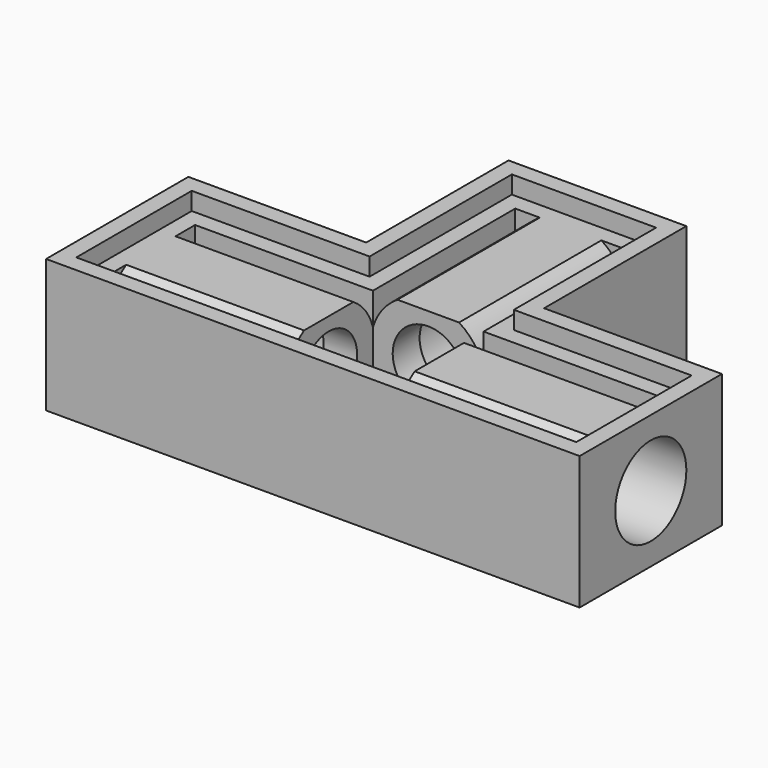
from build123d import *

# Parameters (mm, degrees)
F1_DEPTH  = 19.05
F2_T      = -2.4
F4_DEPTH  = 14.11
F5_R      = 8.255
F5_R_2    = 6.35
F5_R_3    = 5.08
F6_DEPTH  = 30.2
F7_DEPTH  = 25.4
F8_DEPTH  = 34.5948
F9_R      = 8.255
F9_R_2    = 6.35
F9_R_3    = 5.08
F10_DEPTH = 30.2
F11_DEPTH = 25.4
F12_DEPTH = 36.9316
F13_R     = 8.255
F13_R_2   = 6.35
F13_R_3   = 5.08
F14_DEPTH = 30.2
F15_DEPTH = 25.4
F16_DEPTH = 31.242
F17_W     = 3.7311392443
F17_H     = 25.4
F17_W_2   = 25.4
F17_H_2   = 3.7311392443
F20_DEPTH = 2.54


with BuildPart() as f1:
    # F0 (on Top) → F1 (new body)
    with BuildSketch(Plane.XY):
        Polygon((-12.7, 25.4), (-38.1, 25.4), (-38.1, 0), (38.1, 0), (38.1, 25.4), (12.7, 25.4), (12.7, 50.8), (-12.7, 50.8), align=None)
    extrude(amount=F1_DEPTH)

    # F2
    f2_openings = [f1.faces().sort_by_distance(p)[0] for p in [
        (0, 19.05, 19.05),
    ]]
    offset(amount=F2_T, openings=f2_openings, kind=Kind.INTERSECTION)

    # F3 (on face) → F4 (join, through all)
    with BuildSketch(Plane.XY.offset(2.4)):
        Polygon((10.3, 48.4), (-10.3, 48.4), (-10.3, 23), (-35.7, 23), (-35.7, 2.4), (35.7, 2.4), (35.7, 23), (10.3, 23), align=None)
        Polygon((-33.3, 4.8), (-33.3, 20.6), (-7.9, 20.6), (-7.9, 46), (7.9, 46), (7.9, 20.6), (33.3, 20.6), (33.3, 4.8), align=None, mode=Mode.SUBTRACT)
    extrude(amount=F4_DEPTH)

    # F5 (on face) → F6 (join, through all)
    with BuildSketch(Plane(origin=(0, 50.8, 0), x_dir=(-1, 0, 0), z_dir=(0, 1, 0))):
        with Locations((0, 9.525)):
            Circle(F5_R)
        with Locations((0, 9.525)):
            Circle(F5_R_2, mode=Mode.SUBTRACT)
        with Locations((0, 9.525)):
            Circle(F5_R_2)
        with Locations((0, 9.525)):
            Circle(F5_R_3, mode=Mode.SUBTRACT)
        with Locations((0, 9.525)):
            Circle(F5_R_3)
    extrude(amount=-F6_DEPTH)

    # F5 (on face) → F7 (cut)
    with BuildSketch(Plane(origin=(0, 50.8, 0), x_dir=(-1, 0, 0), z_dir=(0, 1, 0))):
        with Locations((0, 9.525)):
            Circle(F5_R_2)
        with Locations((0, 9.525)):
            Circle(F5_R_3, mode=Mode.SUBTRACT)
        with Locations((0, 9.525)):
            Circle(F5_R_3)
    extrude(amount=-F7_DEPTH, mode=Mode.SUBTRACT)

    # F5 (on face) → F8 (cut)
    with BuildSketch(Plane(origin=(0, 50.8, 0), x_dir=(-1, 0, 0), z_dir=(0, 1, 0))):
        with Locations((0, 9.525)):
            Circle(F5_R_3)
    extrude(amount=-F8_DEPTH, mode=Mode.SUBTRACT)

    # F9 (on face) → F10 (join, through all)
    with BuildSketch(Plane.YZ.offset(38.1)):
        with Locations((12.7, 9.525)):
            Circle(F9_R)
        with Locations((12.7, 9.525)):
            Circle(F9_R_2, mode=Mode.SUBTRACT)
        with Locations((12.7, 9.525)):
            Circle(F9_R_2)
        with Locations((12.7, 9.525)):
            Circle(F9_R_3, mode=Mode.SUBTRACT)
        with Locations((12.7, 9.525)):
            Circle(F9_R_3)
    extrude(amount=-F10_DEPTH)

    # F9 (on face) → F11 (cut)
    with BuildSketch(Plane.YZ.offset(38.1)):
        with Locations((12.7, 9.525)):
            Circle(F9_R_2)
        with Locations((12.7, 9.525)):
            Circle(F9_R_3, mode=Mode.SUBTRACT)
    extrude(amount=-F11_DEPTH, mode=Mode.SUBTRACT)

    # F9 (on face) → F12 (cut)
    with BuildSketch(Plane.YZ.offset(38.1)):
        with Locations((12.7, 9.525)):
            Circle(F9_R_3)
    extrude(amount=-F12_DEPTH, mode=Mode.SUBTRACT)

    # F13 (on face) → F14 (join, through all)
    with BuildSketch(Plane(origin=(-38.1, 0, 0), x_dir=(0, -1, 0), z_dir=(-1, 0, 0))):
        with Locations((-12.7, 9.525)):
            Circle(F13_R)
        with Locations((-12.7, 9.525)):
            Circle(F13_R_2, mode=Mode.SUBTRACT)
        with Locations((-12.7, 9.525)):
            Circle(F13_R_2)
        with Locations((-12.7, 9.525)):
            Circle(F13_R_3, mode=Mode.SUBTRACT)
        with Locations((-12.7, 9.525)):
            Circle(F13_R_3)
    extrude(amount=-F14_DEPTH)

    # F13 (on face) → F15 (cut)
    with BuildSketch(Plane(origin=(-38.1, 0, 0), x_dir=(0, -1, 0), z_dir=(-1, 0, 0))):
        with Locations((-12.7, 9.525)):
            Circle(F13_R_2)
        with Locations((-12.7, 9.525)):
            Circle(F13_R_3, mode=Mode.SUBTRACT)
        with Locations((-12.7, 9.525)):
            Circle(F13_R_3)
    extrude(amount=-F15_DEPTH, mode=Mode.SUBTRACT)

    # F13 (on face) → F16 (cut)
    with BuildSketch(Plane(origin=(-38.1, 0, 0), x_dir=(0, -1, 0), z_dir=(-1, 0, 0))):
        with Locations((-12.7, 9.525)):
            Circle(F13_R_3)
    extrude(amount=-F16_DEPTH, mode=Mode.SUBTRACT)

    # F17 (on face) → F18 (join, up to the next surface of F1)
    with BuildSketch(Plane.XY.offset(2.4)):
        with Locations((-6.0344303778, 33.3)):
            Rectangle(F17_W, F17_H)
        with Locations((-20.6, 18.7344303778)):
            Rectangle(F17_W_2, F17_H_2)
        with Locations((6.0344303778, 33.3)):
            Rectangle(F17_W, F17_H)
        with Locations((-20.6, 6.6655696222)):
            Rectangle(F17_W_2, F17_H_2)
        with Locations((20.6, 18.7344303778)):
            Rectangle(F17_W_2, F17_H_2)
        with Locations((20.6, 6.6655696222)):
            Rectangle(F17_W_2, F17_H_2)
    extrude(until=Until.NEXT)

    # F19 (on face) → F20 (cut, through all)
    with BuildSketch(Plane.XY.offset(19.05)):
        Polygon((-10.3, 23), (-35.7, 23), (-35.7, 2.4), (35.7, 2.4), (35.7, 23), (10.3, 23), (10.3, 48.4), (-10.3, 48.4), align=None)
        Polygon((7.9, 46), (7.9, 20.6), (33.3, 20.6), (33.3, 17.0994090512), (33.3, 8.3005909488), (33.3, 4.8), (7.9, 4.8), (-7.9, 4.8), (-33.3, 4.8), (-33.3, 8.3005909488), (-33.3, 17.0994090512), (-33.3, 20.6), (-7.9, 20.6), (-7.9, 46), (-4.3994090512, 46), (4.3994090512, 46), align=None, mode=Mode.SUBTRACT)
        Polygon((-7.9, 20.6), (7.9, 20.6), (7.9, 46), (4.3994090512, 46), (-4.3994090512, 46), (-7.9, 46), align=None)
        Polygon((-7.9, 4.8), (-7.9, 20.6), (-33.3, 20.6), (-33.3, 17.0994090512), (-33.3, 8.3005909488), (-33.3, 4.8), align=None)
        Polygon((33.3, 20.6), (7.9, 20.6), (7.9, 4.8), (33.3, 4.8), (33.3, 8.3005909488), (33.3, 17.0994090512), align=None)
    extrude(amount=-F20_DEPTH, mode=Mode.SUBTRACT)


solid = f1.part
